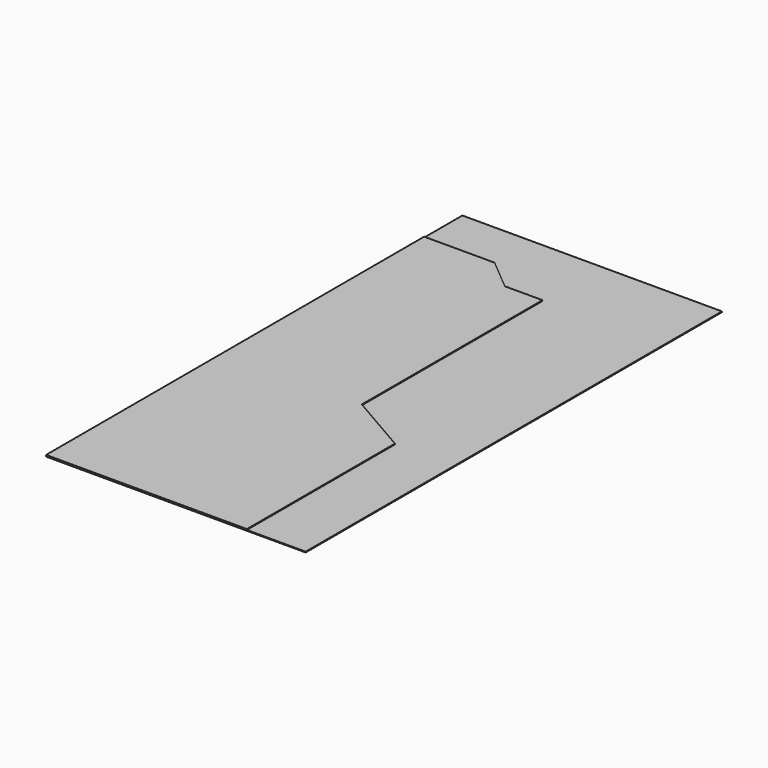
from build123d import *

# Parameters (mm, degrees)
F3_DEPTH = 25
F5_DEPTH = 25


# Not quite as in the source:
# - the program builds the solid bodies; features that only make, move or delete a surface that nothing else refers to are left out


with BuildPart() as f3:
    # F0 (on Top) → F3 (new body)
    with BuildSketch(Plane.XY):
        Polygon((-2250, 3961.3792896271), (-2250, 2435.6238925925), (0, 2435.6238925925), (995.8577760547, 1600), (2195.8577760547, 1600), (2195.8577760547, 600), (2195.8577760547, 0), (2195.8577760547, -5610), (4161.7354426453, -6745), (4161.7354426453, -12655), (6038.0616188049, -12655), (6038.0616188049, 3961.3792896271), align=None)
        Polygon((0, 2435.6238925925), (-2250, 2435.6238925925), (-2250, -12655), (4161.7354426453, -12655), (4161.7354426453, -6745), (2195.8577760547, -5610), (2195.8577760547, 0), (2195.8577760547, 600), (2195.8577760547, 1600), (995.8577760547, 1600), align=None)
    extrude(amount=-F3_DEPTH)

    # F0 (on Top) → F5 (join)
    with BuildSketch(Plane.XY):
        Polygon((0, 2435.6238925925), (-2250, 2435.6238925925), (-2250, -12655), (4161.7354426453, -12655), (4161.7354426453, -6745), (2195.8577760547, -5610), (2195.8577760547, 0), (2195.8577760547, 600), (2195.8577760547, 1600), (995.8577760547, 1600), align=None)
    extrude(amount=F5_DEPTH)


solid = f3.part
